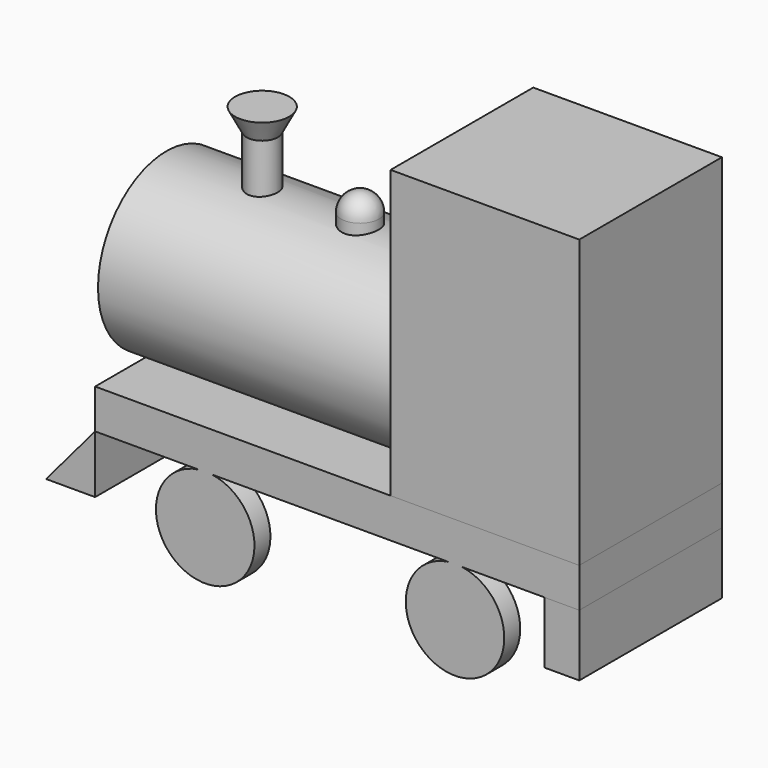
from build123d import *

# Parameters (mm, degrees)
F0_W      = 98.6387990415
F0_H      = 8.0412067473
F1_DEPTH  = 18.161
F2_R      = 17.4226132222
F3_DEPTH  = 60.198
F4_W      = 36.322
F4_H      = 58.4327615798
F5_DEPTH  = 38.4407990415
F8_R      = 10.0363069499
F9_DEPTH  = 4.064
F12_DEPTH = 36.322
F15_W     = 7.0395842195
F15_H     = 12.5978905708
F16_DEPTH = 36.322
F17_W     = 10.1855276152
F17_H     = 10.1855276152
F18_DEPTH = 2.54


with BuildPart() as f1:
    # F0 (on Front) → F1 (new body, symmetric)
    with BuildSketch(Plane.XZ):
        with Locations((2.2148583084, -15.412312001)):
            Rectangle(F0_W, F0_H)
    extrude(amount=F1_DEPTH, both=True)

    # F8 (on face) → F9 (join)
    with BuildSketch(Plane(origin=(0, 18.161, 0), x_dir=(-1, 0, 0), z_dir=(0, 1, 0))):
        with Locations((24.6769684583, -29.3797980994)):
            Circle(F8_R)
        with Locations((-26.2185372412, -29.3797980994)):
            Circle(F8_R)
    extrude(amount=-F9_DEPTH)


with BuildPart() as f3:
    # F2 (on face) → F3 (new body)
    with BuildSketch(Plane(origin=(-47.1045412123, 0, 0), x_dir=(0, -1, 0), z_dir=(-1, 0, 0))):
        with Locations((0, 6.0309045948)):
            Circle(F2_R)
    extrude(amount=-F3_DEPTH)

    # F6 (on Front) → F7 (revolve)
    with BuildSketch(Plane.XZ):
        Polygon((-27.5913029909, 37.7604365349), (-27.5913029909, 18.1952826679), (-24.3897307664, 18.1952826679), (-24.3897307664, 33.3138108253), (-22.0774877816, 37.7604365349), align=None)
    revolve(axis=Axis((-27.5913029909, 0, 33.3138089627), (0, 0, 1)))

    # F13 (on Front) → F14 (revolve)
    with BuildSketch(Plane.XZ):
        with BuildLine():
            Line((-7.6616099104, 29.1813736411), (-7.6616099104, 17.1943176538))
            Line((-7.6616099104, 17.1943176538), (-3.8142945988, 17.1943176538))
            Line((-3.8142945988, 17.1943176538), (-3.8142945988, 25.3340583295))
            ThreePointArc((-3.8142945988, 25.3340583295), (-4.9411471642, 28.0545210757), (-7.6616099104, 29.1813736411))
        make_face()
    revolve(axis=Axis((-7.6616099104, 0, 29.9853375182), (0, 0, 1)))

    # F17 (on face) → F18 (join)
    with BuildSketch(Plane(origin=(-47.1045412123, 0, 0), x_dir=(0, -1, 0), z_dir=(-1, 0, 0))):
        with Locations((0, 6.0309045948)):
            Rectangle(F17_W, F17_H)
    extrude(amount=F18_DEPTH)


with BuildPart() as f5:
    # F4 (on face) → F5 (new body, through all)
    with BuildSketch(Plane.YZ.offset(13.0934587877)):
        with Locations((0, 17.8246721625)):
            Rectangle(F4_W, F4_H)
    extrude(amount=F5_DEPTH)


with BuildPart() as f10_1:
    # F10: instance of F1
    add(f1.part.mirror(Plane.XZ))


with BuildPart() as f12:
    # F11 (on face) → F12 (new body, through all)
    with BuildSketch(Plane(origin=(0, 18.161, 0), x_dir=(-1, 0, 0), z_dir=(0, 1, 0))):
        Polygon((57.0925623178, -31.226683408), (47.1045412123, -19.4329153746), (47.1045412123, -31.226683408), align=None)
    extrude(amount=-F12_DEPTH)


with BuildPart() as f16:
    # F15 (on face) → F16 (new body, through all)
    with BuildSketch(Plane(origin=(0, 18.161, 0), x_dir=(-1, 0, 0), z_dir=(0, 1, 0))):
        with Locations((-48.0144657195, -25.73186066)):
            Rectangle(F15_W, F15_H)
    extrude(amount=-F16_DEPTH)


solid = Compound([f1.part, f3.part, f5.part, f10_1.part, f12.part, f16.part])
